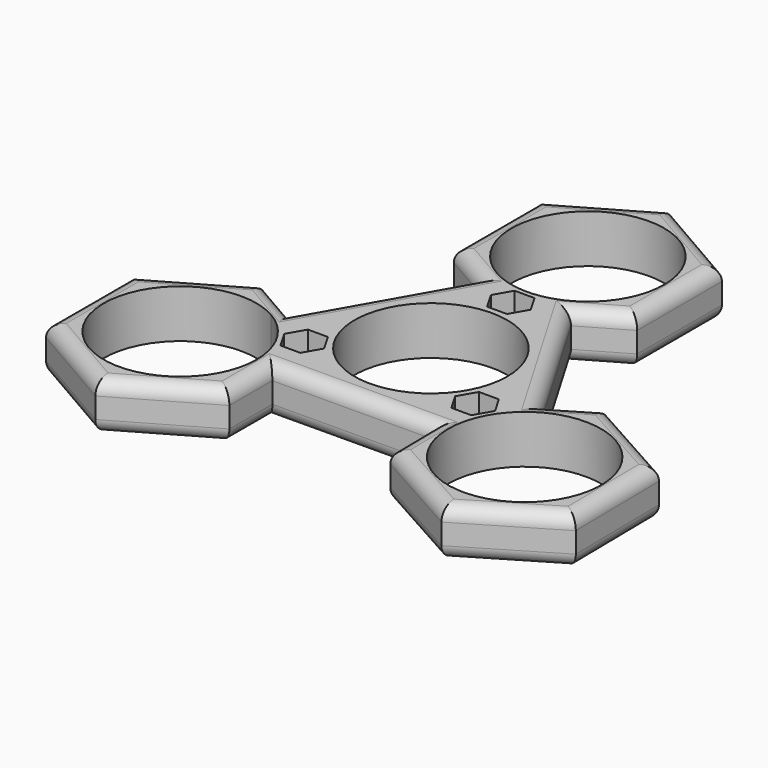
from build123d import *

# Parameters (mm, degrees)
F0_R     = 11.075
F1_DEPTH = 7
F2_R     = 2
F4_DEPTH = 25


# Not quite as in the source:
# - a feature names something its author has since deleted; it is built from what else it names


with BuildPart() as f1:
    # F0 (on Top) → F1 (new body)
    with BuildSketch(Plane.XY):
        with BuildLine():
            ThreePointArc((10.8590541373, 28.4748429105), (9.3936805028, 22.9693269387), (5.3853374572, 18.9207207546))
            Line((5.3853374572, 18.9207207546), (6.5097166395, 17.0028645343))
            Line((6.5097166395, 17.0028645343), (13.0819100939, 20.7973221943))
            Line((13.0819100939, 20.7973221943), (13.0819100939, 36.1523636266))
            Line((13.0819100939, 36.1523636266), (-0.2159458627, 43.8298843428))
            Line((-0.2159458627, 43.8298843428), (-13.5138018192, 36.1523636266))
            Line((-13.5138018192, 36.1523636266), (-13.5138018192, 20.7973221943))
            Line((-13.5138018192, 20.7973221943), (-6.7881393171, 16.9142591382))
            Line((-6.7881393171, 16.9142591382), (-5.6894167006, 18.8469281837))
            ThreePointArc((-5.6894167006, 18.8469281837), (-5.7853684301, 38.0475727858), (10.8590541373, 28.4748429105))
        make_face()
        with BuildLine():
            Line((6.5097166395, 17.0028645343), (5.3853374572, 18.9207207546))
            ThreePointArc((5.3853374572, 18.9207207546), (-0.1421532918, 17.4000887526), (-5.6894167006, 18.8469281837))
            Line((-5.6894167006, 18.8469281837), (-6.7881393171, 16.9142591382))
            Line((-6.7881393171, 16.9142591382), (-0.2159458627, 13.1198014782))
            Line((-0.2159458627, 13.1198014782), (6.5097166395, 17.0028645343))
        make_face()
        Polygon((18.1892172392, -2.9188871567), (6.5097166395, 17.0028645343), (-0.2159458627, 13.1198014782), (-6.7881393171, 16.9142591382), (-18.2011320695, -3.1613609301), (-11.4686565798, -7.0562964045), (-11.4753544728, -14.6335356233), (11.6169113166, -14.4796687622), (11.5092421808, -6.9031915863), align=None)
        with Locations((-0.0247963396, -0.2127871583)):
            Circle(F0_R, mode=Mode.SUBTRACT)
        with BuildLine():
            Line((19.313711516, -4.836939694), (18.1892172392, -2.9188871567))
            Line((18.1892172392, -2.9188871567), (11.5092421808, -6.9031915863))
            Line((11.5092421808, -6.9031915863), (11.6169113166, -14.4796687622))
            Line((11.6169113166, -14.4796687622), (13.840240678, -14.4648544208))
            ThreePointArc((13.840240678, -14.4648544208), (15.2870801091, -8.917591012), (19.313711516, -4.836939694))
        make_face()
        with BuildLine():
            Line((-11.4686565798, -7.0562964045), (-18.2011320695, -3.1613609301))
            Line((-18.2011320695, -3.1613609301), (-19.2999671542, -5.0942278088))
            ThreePointArc((-19.2999671542, -5.0942278088), (-15.2193158362, -9.1208592157), (-13.6986838342, -14.6483499647))
            Line((-13.6986838342, -14.6483499647), (-11.4753544728, -14.6335356233))
            Line((-11.4753544728, -14.6335356233), (-11.4686565798, -7.0562964045))
        make_face()
        with BuildLine():
            Line((-19.2999671542, -5.0942278088), (-18.2011320695, -3.1613609301))
            Line((-18.2011320695, -3.1613609301), (-24.759864777, 0.6330592247))
            Line((-24.759864777, 0.6330592247), (-38.0646461892, -7.0327869064))
            Line((-38.0646461892, -7.0327869064), (-38.0782194043, -22.3879886667))
            Line((-38.0782194043, -22.3879886667), (-24.7870112072, -30.077344296))
            Line((-24.7870112072, -30.077344296), (-11.4822297949, -22.4114981649))
            Line((-11.4822297949, -22.4114981649), (-11.4753544728, -14.6335356233))
            Line((-11.4753544728, -14.6335356233), (-13.6986838342, -14.6483499647))
            ThreePointArc((-13.6986838342, -14.6483499647), (-13.6984994528, -14.6852460454), (-13.6984379921, -14.7221425356))
            ThreePointArc((-13.6984379921, -14.7221425356), (-34.3461678674, -20.2915651031), (-19.2999671542, -5.0942278088))
        make_face()
        with BuildLine():
            Line((24.6968043769, 0.9625956381), (18.1892172392, -2.9188871567))
            Line((18.1892172392, -2.9188871567), (19.313711516, -4.836939694))
            ThreePointArc((19.313711516, -4.836939694), (30.4205108077, -4.7814354844), (35.9899948359, -14.3910618499))
            ThreePointArc((35.9899948359, -14.3910618499), (24.9518913261, -25.4660003892), (13.840240678, -14.4648544208))
            Line((13.840240678, -14.4648544208), (11.6169113166, -14.4796687622))
            Line((11.6169113166, -14.4796687622), (11.7274326398, -22.2568490742))
            Line((11.7274326398, -22.2568490742), (25.1331852948, -29.7447193378))
            Line((25.1331852948, -29.7447193378), (38.3207474909, -21.8789321135))
            Line((38.3207474909, -21.8789321135), (38.1025570319, -6.5252746256))
            Line((38.1025570319, -6.5252746256), (24.6968043769, 0.9625956381))
        make_face()
    extrude(amount=F1_DEPTH)

    # F2
    f2_edges = [f1.edges().sort_by_distance(p)[0] for p in [
        (-10.150971, 18.855791, 7),
        (-13.513802, 28.474843, 7),
        (-6.864874, 39.991124, 7),
        (6.432982, 39.991124, 7),
        (13.08191, 28.474843, 7),
        (12.349467, 7.041989, 7),
        (9.795813, 18.900093, 7),
        (21.443011, -0.978146, 7),
        (31.399681, -2.781339, 7),
        (38.211652, -14.202103, 7),
        (31.726966, -25.811826, 7),
        (18.430309, -26.000784, 7),
        (11.672172, -18.368259, 7),
        (0.070778, -14.556602, 7),
        (-11.478792, -18.522517, 7),
        (-31.432615, -26.232666, 7),
        (-18.134621, -26.244421, 7),
        (-38.071433, -14.710388, 7),
        (-31.412255, -3.199864, 7),
        (-21.480498, -1.264151, 7),
        (-12.494636, 6.876449, 7),
        (31.726966, -25.811826, 0),
        (38.211652, -14.202103, 0),
        (31.399681, -2.781339, 0),
        (21.443011, -0.978146, 0),
        (18.430309, -26.000784, 0),
        (11.672172, -18.368259, 0),
        (12.349467, 7.041989, 0),
        (0.070778, -14.556602, 0),
        (9.795813, 18.900093, 0),
        (13.08191, 28.474843, 0),
        (6.432982, 39.991124, 0),
        (-6.864874, 39.991124, 0),
        (-13.513802, 28.474843, 0),
        (-10.150971, 18.855791, 0),
        (-12.494636, 6.876449, 0),
        (-21.480498, -1.264151, 0),
        (-31.412255, -3.199864, 0),
        (-38.071433, -14.710388, 0),
        (-31.432615, -26.232666, 0),
        (-18.134621, -26.244421, 0),
        (-11.478792, -18.522517, 0),
    ]]
    fillet(f2_edges, radius=F2_R)

    # F3 (on face) → F4 (cut)
    with BuildSketch(Plane.XY.offset(7)):
        Polygon((1.443375673, 16.7368283158), (-1.443375673, 16.7368283158), (-2.8867513459, 14.2368283158), (-1.443375673, 11.7368283158), (1.443375673, 11.7368283158), (2.8867513459, 14.2368283158), align=None)
        Polygon((-10.8739663642, -5.3167335935), (-13.7607177101, -5.3167335935), (-15.2040933831, -7.8167335935), (-13.7607177101, -10.3167335935), (-10.8739663642, -10.3167335935), (-9.4305906912, -7.8167335935), align=None)
        Polygon((13.7978978307, -5.1664386955), (10.9111464847, -5.1664386955), (9.4677708117, -7.6664386955), (10.9111464847, -10.1664386955), (13.7978978307, -10.1664386955), (15.2412735036, -7.6664386955), align=None)
    extrude(amount=-F4_DEPTH, mode=Mode.SUBTRACT)


solid = f1.part
